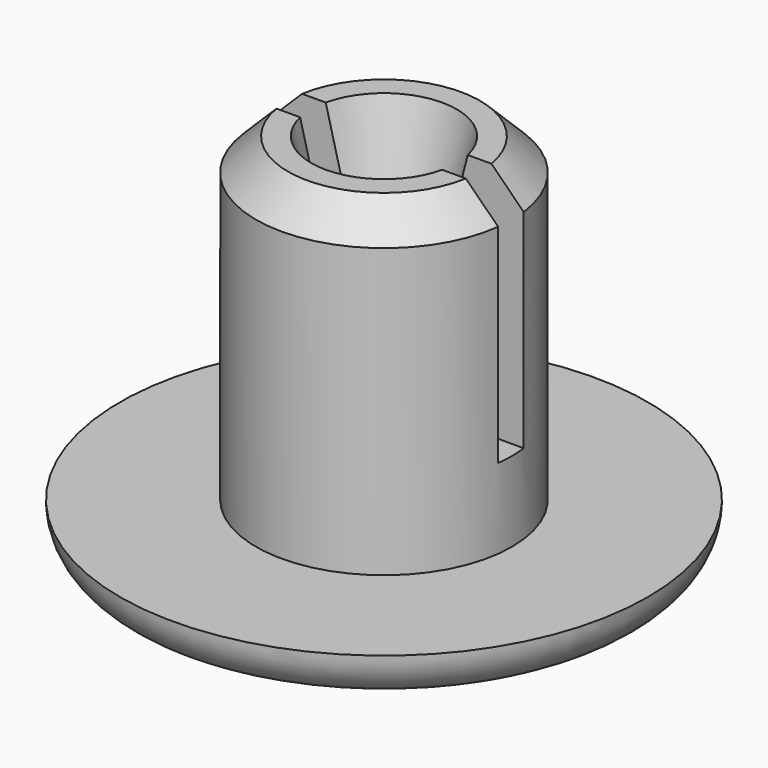
from build123d import *

# Parameters (mm, degrees)
F0_R      = 16.5
F1_DEPTH  = 3
F2_R      = 8
F3_DEPTH  = 20
F4_R      = 2.55
F5_DEPTH  = 25
F6_R      = 4.5
F7_DEPTH  = 5
F8_W      = 17.7715833097
F8_H      = 2
F9_DEPTH  = 15
F10_R     = 2.99999
F11_SIZE  = 2
F12_SIZE2 = 2
F12_SIZE  = 8


# Not quite as in the source:
# - a fillet or chamfer is up to 0.001 mm smaller than in the source, because OpenCascade refuses the exact size


with BuildPart() as f1:
    # F0 (on Top) → F1 (new body)
    with BuildSketch(Plane.XY):
        Circle(F0_R)
    extrude(amount=F1_DEPTH)

    # F2 (on face) → F3 (join)
    with BuildSketch(Plane.XY.offset(3)):
        Circle(F2_R)
    extrude(amount=F3_DEPTH)

    # F4 (on face) → F5 (cut)
    with BuildSketch(Plane(origin=(0, 0, 0), x_dir=(1, 0, 0), z_dir=(0, 0, -1))):
        Circle(F4_R)
    extrude(amount=-F5_DEPTH, mode=Mode.SUBTRACT)

    # F6 (on face) → F7 (cut)
    with BuildSketch(Plane(origin=(0, 0, 0), x_dir=(1, 0, 0), z_dir=(0, 0, -1))):
        Circle(F6_R)
    extrude(amount=-F7_DEPTH, mode=Mode.SUBTRACT)

    # F8 (on face) → F9 (cut)
    with BuildSketch(Plane.XY.offset(23)):
        Rectangle(F8_W, F8_H)
    extrude(amount=-F9_DEPTH, mode=Mode.SUBTRACT)

    # F10 (radius 3 in the source; OpenCascade refuses exactly that, so slightly less here)
    f10_edges = [f1.edges().sort_by_distance(p)[0] for p in [
        (-16.5, 0, 0),
    ]]
    fillet(f10_edges, radius=F10_R)

    # F11
    f11_edges = [f1.edges().sort_by_distance(p)[0] for p in [
        (0, 8, 23),
        (0, -8, 23),
    ]]
    chamfer(f11_edges, length=F11_SIZE)

    # F12
    f12_edges = [f1.edges().sort_by_distance(p)[0] for p in [
        (0, 2.55, 23),
        (0, -2.55, 23),
    ]]
    f12_side = f1.faces().sort_by_distance((2.498413, 0.510324, 7.806088))[0]
    chamfer(f12_edges, length=F12_SIZE, length2=F12_SIZE2, reference=f12_side)


solid = f1.part
